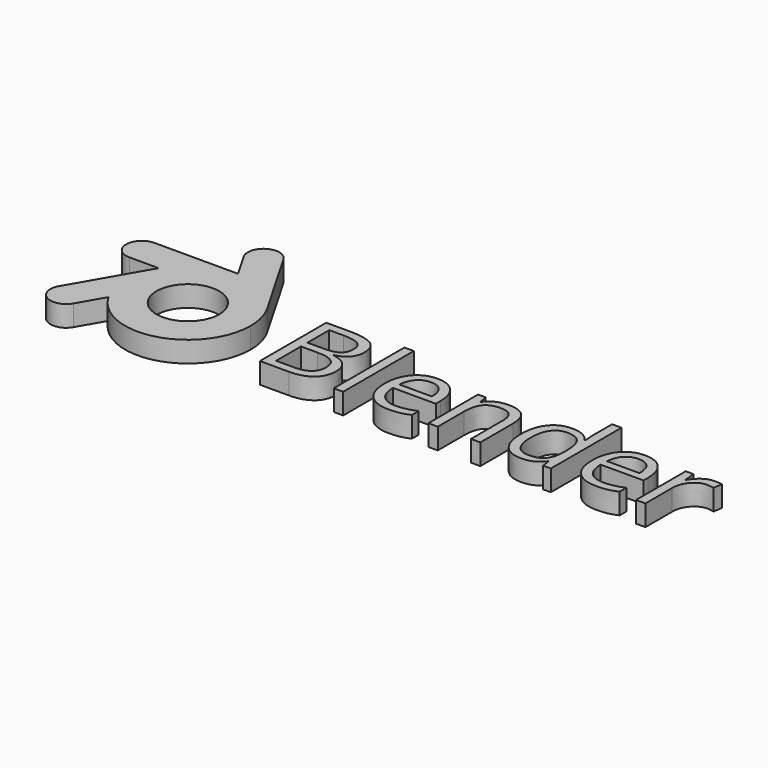
from build123d import *

# Parameters (mm, degrees)
F1_DEPTH     = 25.4
F2_TEXT_SIZE = 141.1111111111
F3_DEPTH     = 25.4


# Not quite as in the source:
# - Text() gives the source's letters only with a copy of the font that has no kerning and outlines rounded to 1/6400 em; it was checked with that copy


with BuildPart() as f1:
    # F0 (on Top) → F1 (new body)
    with BuildSketch(Plane.XY):
        with BuildLine():
            ThreePointArc((0, 76.2), (38.1, 65.9911357684), (65.9911357684, 38.1))
            Line((65.9911357684, 38.1), (15.1911357684, 126.0881810245))
            ThreePointArc((15.1911357684, 126.0881810245), (-10.8316481737, 133.0609649666), (-17.8044321158, 107.0381810245))
            Line((-17.8044321158, 107.0381810245), (0, 76.2))
        make_face()
        with BuildLine():
            ThreePointArc((-65.9911357684, -38.1), (19.7220112368, -73.6035479632), (76.2, 0))
            ThreePointArc((76.2, 0), (73.6035479632, 19.7220112368), (65.9911357684, 38.1))
            ThreePointArc((65.9911357684, 38.1), (38.1, 65.9911357684), (0, 76.2))
            Line((0, 76.2), (32.9955678842, 19.05))
            ThreePointArc((32.9955678842, 19.05), (36.8017739816, 9.8610056184), (38.1, 0))
            ThreePointArc((38.1, 0), (-9.8610056184, -36.8017739816), (-32.9955678842, 19.05))
            Line((-32.9955678842, 19.05), (-65.9911357684, -38.1))
        make_face()
        with BuildLine():
            ThreePointArc((-65.9911357684, 38.1), (-76.2, 0), (-65.9911357684, -38.1))
            Line((-65.9911357684, -38.1), (-32.9955678842, 19.05))
            ThreePointArc((-32.9955678842, 19.05), (-19.05, 32.9955678842), (0, 38.1))
            Line((0, 38.1), (-65.9911357684, 38.1))
        make_face()
        with BuildLine():
            Line((32.9955678842, 19.05), (0, 76.2))
            ThreePointArc((0, 76.2), (-38.1, 65.9911357684), (-65.9911357684, 38.1))
            Line((-65.9911357684, 38.1), (0, 38.1))
            ThreePointArc((0, 38.1), (19.05, 32.9955678842), (32.9955678842, 19.05))
        make_face()
        with BuildLine():
            Line((-83.7955678842, -68.9381810245), (-65.9911357684, -38.1))
            ThreePointArc((-65.9911357684, -38.1), (-76.2, 0), (-65.9911357684, 38.1))
            Line((-65.9911357684, 38.1), (-116.7911357684, -49.8881810245))
            ThreePointArc((-116.7911357684, -49.8881810245), (-109.8183518263, -75.9109649666), (-83.7955678842, -68.9381810245))
        make_face()
        with BuildLine():
            ThreePointArc((-65.9911357684, 38.1), (-38.1, 65.9911357684), (0, 76.2))
            Line((0, 76.2), (-101.6, 76.2))
            ThreePointArc((-101.6, 76.2), (-120.65, 57.15), (-101.6, 38.1))
            Line((-101.6, 38.1), (-65.9911357684, 38.1))
        make_face()
    extrude(amount=F1_DEPTH)


with BuildPart() as f3:
    # F2 (on Top) → F3 (new body)
    with BuildSketch(Plane.XY):
        with Locations((114.3, -50.8)):
            Text('Blender', F2_TEXT_SIZE, font='Open Sans', text_align=(TextAlign.LEFT, TextAlign.BOTTOM))
    extrude(amount=F3_DEPTH)


solid = Compound([f1.part, f3.part])
